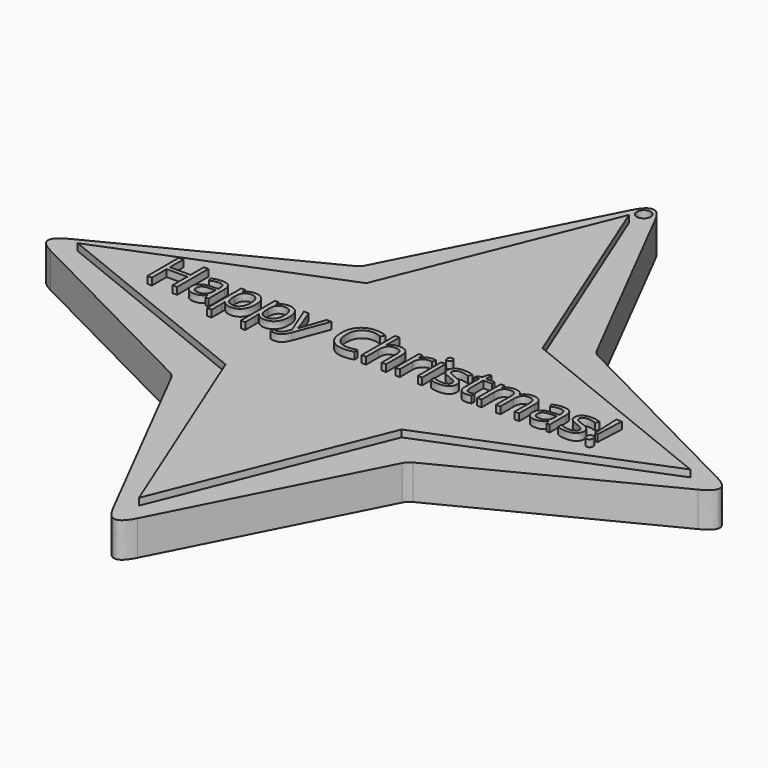
from build123d import *

# Parameters (mm, degrees)
F0_R         = 1
F1_DEPTH     = 5
F2_DEPTH     = 6
F3_DEPTH     = 1
F4_T1_DEPTH  = 5
F4_T3_DEPTH  = 24.6074090806
F5_TEXT_SIZE = 7.8890974948
F6_DEPTH     = 1


# Not quite as in the source:
# - a fillet or chamfer that OpenCascade refuses, or shapes differently, is made with other operations: its cross-section is extruded or revolved along the edge and cut away or added
# - Text() gives the source's letters only with a copy of the font that has no kerning and outlines rounded to 1/6400 em; it was checked with that copy


with BuildPart() as f1:
    # F0 (on Top) → F1 (new body)
    with BuildSketch(Plane.XY):
        Polygon((16.8876647949, 16.8876647949), (0, 50), (-16.8876647949, 16.8876647949), (-50, 0), (-16.8876647949, -16.8876647949), (0, -50), (16.8876647949, -16.8876647949), (50, 0), align=None)
        Polygon((-12.6450241078, 12.6450241078), (0, 44), (12.6450241078, 12.6450241078), (44, 0), (12.6450241078, -12.6450241078), (0, -44), (-12.6450241078, -12.6450241078), (-44, 0), align=None, mode=Mode.SUBTRACT)
        with Locations((0, 46.6435588896)):
            Circle(F0_R, mode=Mode.SUBTRACT)
        Polygon((12.6450241078, 12.6450241078), (0, 44), (-12.6450241078, 12.6450241078), (-44, 0), (-12.6450241078, -12.6450241078), (0, -44), (12.6450241078, -12.6450241078), (44, 0), align=None)
    extrude(amount=F1_DEPTH)

    # F0 (on Top) → F2 (join)
    with BuildSketch(Plane.XY):
        Polygon((12.6450241078, 12.6450241078), (0, 44), (-12.6450241078, 12.6450241078), (-44, 0), (-12.6450241078, -12.6450241078), (0, -44), (12.6450241078, -12.6450241078), (44, 0), align=None)
    extrude(amount=F2_DEPTH)

    # F0 (on Top) → F3 (join)
    with BuildSketch(Plane.XY):
        Polygon((12.6450241078, 12.6450241078), (0, 44), (-12.6450241078, 12.6450241078), (-44, 0), (-12.6450241078, -12.6450241078), (0, -44), (12.6450241078, -12.6450241078), (44, 0), align=None)
    extrude(amount=-F3_DEPTH)

    # F4: fillet of radius 2 on 8 edges, made by hand

    # F4_s2 → F4_t1 (join)
    with BuildSketch(Plane.XY):
        with BuildLine():
            add(Edge.make_bspline(
                [(17.46580262, 16.5928079769), (16.8876647949, 16.8876647949), (16.5928079769, 17.46580262)],
                knots=[0, 0, 0, 1, 1, 1], degree=2, weights=[1, 1, 1]))
            Line((16.5928079769, 17.46580262), (16.8876647949, 16.8876647949))
            Line((16.8876647949, 16.8876647949), (17.46580262, 16.5928079769))
        make_face()
        with BuildLine():
            add(Edge.make_bspline(
                [(-16.5928079769, -17.46580262), (-16.8876647949, -16.8876647949), (-17.46580262, -16.5928079769)],
                knots=[0, 0, 0, 1, 1, 1], degree=2, weights=[1, 1, 1]))
            Line((-17.46580262, -16.5928079769), (-16.8876647949, -16.8876647949))
            Line((-16.8876647949, -16.8876647949), (-16.5928079769, -17.46580262))
        make_face()
        with BuildLine():
            add(Edge.make_bspline(
                [(-16.5928079769, 17.46580262), (-16.8876647949, 16.8876647949), (-17.46580262, 16.5928079769)],
                knots=[0, 0, 0, 1, 1, 1], degree=2, weights=[1, 1, 1]))
            Line((-17.46580262, 16.5928079769), (-16.8876647949, 16.8876647949))
            Line((-16.8876647949, 16.8876647949), (-16.5928079769, 17.46580262))
        make_face()
        with BuildLine():
            add(Edge.make_bspline(
                [(17.46580262, -16.5928079769), (16.8876647949, -16.8876647949), (16.5928079769, -17.46580262)],
                knots=[0, 0, 0, 1, 1, 1], degree=2, weights=[1, 1, 1]))
            Line((16.5928079769, -17.46580262), (16.8876647949, -16.8876647949))
            Line((16.8876647949, -16.8876647949), (17.46580262, -16.5928079769))
        make_face()
    extrude(amount=F4_T1_DEPTH)

    # F4_s4 → F4_t3 (cut)
    with BuildSketch(Plane.XY.offset(-9.8037045403)):
        with BuildLine():
            add(Edge.make_bspline(
                [(1.7816627717, -46.5066209192), (0, -50), (-1.7816627717, -46.5066209192)],
                knots=[0, 0, 0, 1, 1, 1], degree=2, weights=[1, 1, 1]))
            Line((-1.7816627717, -46.5066209192), (0, -50))
            Line((0, -50), (1.7816627717, -46.5066209192))
        make_face()
        with BuildLine():
            add(Edge.make_bspline(
                [(1.7816627717, 46.5066209192), (0, 50), (-1.7816627717, 46.5066209192)],
                knots=[0, 0, 0, 1, 1, 1], degree=2, weights=[1, 1, 1]))
            Line((-1.7816627717, 46.5066209192), (0, 50))
            Line((0, 50), (1.7816627717, 46.5066209192))
        make_face()
        with BuildLine():
            add(Edge.make_bspline(
                [(46.5066209192, -1.7816627717), (50, 0), (46.5066209192, 1.7816627717)],
                knots=[0, 0, 0, 1, 1, 1], degree=2, weights=[1, 1, 1]))
            Line((46.5066209192, 1.7816627717), (50, 0))
            Line((50, 0), (46.5066209192, -1.7816627717))
        make_face()
        with BuildLine():
            add(Edge.make_bspline(
                [(-46.5066209192, -1.7816627717), (-50, 0), (-46.5066209192, 1.7816627717)],
                knots=[0, 0, 0, 1, 1, 1], degree=2, weights=[1, 1, 1]))
            Line((-46.5066209192, 1.7816627717), (-50, 0))
            Line((-50, 0), (-46.5066209192, -1.7816627717))
        make_face()
    extrude(amount=F4_T3_DEPTH, mode=Mode.SUBTRACT)

    # F5 (on face) → F6 (join)
    with BuildSketch(Plane.XY.offset(6)):
        with Locations((-32.5, -2.8400750981)):
            Text('Happy Christmas!', F5_TEXT_SIZE, font='Open Sans', text_align=(TextAlign.LEFT, TextAlign.BOTTOM))
    extrude(amount=F6_DEPTH)


solid = f1.part
